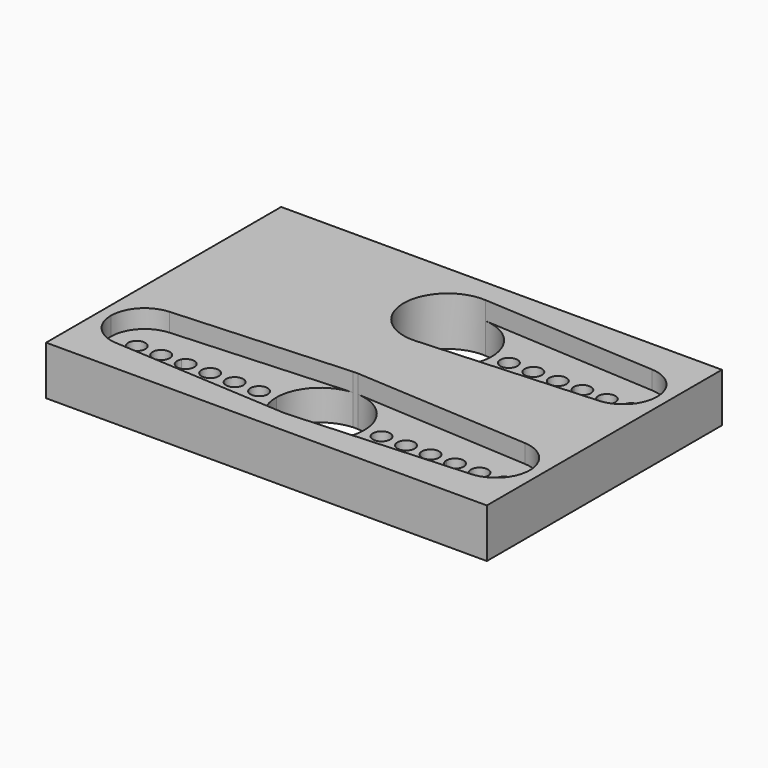
from build123d import *

# Parameters (mm, degrees)
F1_DEPTH = 4
F2_DEPTH = 1.5


with BuildPart() as f1:
    # F0 (on Top) → F1 (new body)
    with BuildSketch(Plane.XY):
        with BuildLine():
            Line((18, 12), (-18, 12))
            Line((-18, 12), (-18, -6.5))
            Line((-18, -6.5), (-17.1, -6.5))
            ThreePointArc((-17.1, -6.5), (-16.3513061937, -4.613926428), (-14.5128919861, -3.7548285662))
            Line((-14.5128919861, -3.7548285662), (-0.2132404181, -2.9063210321))
            ThreePointArc((-0.2132404181, -2.9063210321), (0, -2.9), (0.2132404181, -2.9063210321))
            Line((0.2132404181, -2.9063210321), (14.5128919861, -3.7548285662))
            ThreePointArc((14.5128919861, -3.7548285662), (16.3513061937, -4.613926428), (17.1, -6.5))
            Line((17.1, -6.5), (18, -6.5))
            Line((18, -6.5), (18, 6.5))
            Line((18, 6.5), (18, 12))
        make_face()
        with BuildLine():
            ThreePointArc((14.5128919861, 9.2451714338), (16.3513061937, 8.386073572), (17.1, 6.5))
            ThreePointArc((17.1, 6.5), (16.3513061937, 4.613926428), (14.5128919861, 3.7548285662))
            Line((14.5128919861, 3.7548285662), (0.2132404181, 2.9063210321))
            ThreePointArc((0.2132404181, 2.9063210321), (-3.6, 6.5), (0.2132404181, 10.0936789679))
            Line((0.2132404181, 10.0936789679), (14.5128919861, 9.2451714338))
        make_face(mode=Mode.SUBTRACT)
        with BuildLine():
            Line((-17.1, -6.5), (-18, -6.5))
            Line((-18, -6.5), (-18, -12))
            Line((-18, -12), (18, -12))
            Line((18, -12), (18, -6.5))
            Line((18, -6.5), (17.1, -6.5))
            ThreePointArc((17.1, -6.5), (16.3513061937, -8.386073572), (14.5128919861, -9.2451714338))
            Line((14.5128919861, -9.2451714338), (0.2132404181, -10.0936789679))
            ThreePointArc((0.2132404181, -10.0936789679), (0, -10.1), (-0.2132404181, -10.0936789679))
            Line((-0.2132404181, -10.0936789679), (-14.5128919861, -9.2451714338))
            ThreePointArc((-14.5128919861, -9.2451714338), (-16.3513061937, -8.386073572), (-17.1, -6.5))
        make_face()
        with BuildLine():
            ThreePointArc((-14.5128919861, -3.7548285662), (-16.3513061937, -4.613926428), (-17.1, -6.5))
            Line((-17.1, -6.5), (-15.7, -6.5))
            ThreePointArc((-15.7, -6.5), (-15, -5.8), (-14.3, -6.5))
            Line((-14.3, -6.5), (-13.7, -6.5))
            ThreePointArc((-13.7, -6.5), (-13, -5.8), (-12.3, -6.5))
            Line((-12.3, -6.5), (-11.7, -6.5))
            ThreePointArc((-11.7, -6.5), (-11.6795520913, -6.3320447821), (-11.6194029851, -6.1739019441))
            ThreePointArc((-11.6194029851, -6.1739019441), (-12.5861246414, -4.3902029199), (-14.5128919861, -3.7548285662))
        make_face()
        with BuildLine():
            Line((-15.7, -6.5), (-17.1, -6.5))
            ThreePointArc((-17.1, -6.5), (-16.3513061937, -8.386073572), (-14.5128919861, -9.2451714338))
            ThreePointArc((-14.5128919861, -9.2451714338), (-12.5861246414, -8.6097970801), (-11.6194029851, -6.8260980559))
            ThreePointArc((-11.6194029851, -6.8260980559), (-11.6795520913, -6.6679552179), (-11.7, -6.5))
            Line((-11.7, -6.5), (-12.3, -6.5))
            ThreePointArc((-12.3, -6.5), (-13, -7.2), (-13.7, -6.5))
            Line((-13.7, -6.5), (-14.3, -6.5))
            ThreePointArc((-14.3, -6.5), (-15, -7.2), (-15.7, -6.5))
        make_face()
        with BuildLine():
            Line((-0.2132404181, -2.9063210321), (-14.5128919861, -3.7548285662))
            ThreePointArc((-14.5128919861, -3.7548285662), (-12.5861246414, -4.3902029199), (-11.6194029851, -6.1739019441))
            ThreePointArc((-11.6194029851, -6.1739019441), (-10.8320447821, -5.8204479087), (-10.3, -6.5))
            Line((-10.3, -6.5), (-9.7, -6.5))
            ThreePointArc((-9.7, -6.5), (-9, -5.8), (-8.3, -6.5))
            Line((-8.3, -6.5), (-7.7, -6.5))
            ThreePointArc((-7.7, -6.5), (-7, -5.8), (-6.3, -6.5))
            Line((-6.3, -6.5), (-5.7, -6.5))
            ThreePointArc((-5.7, -6.5), (-5, -5.8), (-4.3, -6.5))
            Line((-4.3, -6.5), (-3.6, -6.5))
            ThreePointArc((-3.6, -6.5), (-2.6198917444, -4.030958233), (-0.2132404181, -2.9063210321))
        make_face()
        with BuildLine():
            ThreePointArc((-11.6194029851, -6.8260980559), (-12.5861246414, -8.6097970801), (-14.5128919861, -9.2451714338))
            Line((-14.5128919861, -9.2451714338), (-0.2132404181, -10.0936789679))
            ThreePointArc((-0.2132404181, -10.0936789679), (-2.6198917444, -8.969041767), (-3.6, -6.5))
            Line((-3.6, -6.5), (-4.3, -6.5))
            ThreePointArc((-4.3, -6.5), (-5, -7.2), (-5.7, -6.5))
            Line((-5.7, -6.5), (-6.3, -6.5))
            ThreePointArc((-6.3, -6.5), (-7, -7.2), (-7.7, -6.5))
            Line((-7.7, -6.5), (-8.3, -6.5))
            ThreePointArc((-8.3, -6.5), (-9, -7.2), (-9.7, -6.5))
            Line((-9.7, -6.5), (-10.3, -6.5))
            ThreePointArc((-10.3, -6.5), (-10.8320447821, -7.1795520913), (-11.6194029851, -6.8260980559))
        make_face()
        with BuildLine():
            Line((0.2132404181, -10.0936789679), (14.5128919861, -9.2451714338))
            ThreePointArc((14.5128919861, -9.2451714338), (12.5861246414, -8.6097970801), (11.6194029851, -6.8260980559))
            ThreePointArc((11.6194029851, -6.8260980559), (10.8320447821, -7.1795520913), (10.3, -6.5))
            Line((10.3, -6.5), (9.7, -6.5))
            ThreePointArc((9.7, -6.5), (9, -7.2), (8.3, -6.5))
            Line((8.3, -6.5), (7.7, -6.5))
            ThreePointArc((7.7, -6.5), (7, -7.2), (6.3, -6.5))
            Line((6.3, -6.5), (5.7, -6.5))
            ThreePointArc((5.7, -6.5), (5, -7.2), (4.3, -6.5))
            Line((4.3, -6.5), (3.6, -6.5))
            ThreePointArc((3.6, -6.5), (2.6198917444, -8.969041767), (0.2132404181, -10.0936789679))
        make_face()
        with BuildLine():
            ThreePointArc((11.6194029851, -6.1739019441), (12.5861246414, -4.3902029199), (14.5128919861, -3.7548285662))
            Line((14.5128919861, -3.7548285662), (0.2132404181, -2.9063210321))
            ThreePointArc((0.2132404181, -2.9063210321), (2.6198917444, -4.030958233), (3.6, -6.5))
            Line((3.6, -6.5), (4.3, -6.5))
            ThreePointArc((4.3, -6.5), (5, -5.8), (5.7, -6.5))
            Line((5.7, -6.5), (6.3, -6.5))
            ThreePointArc((6.3, -6.5), (7, -5.8), (7.7, -6.5))
            Line((7.7, -6.5), (8.3, -6.5))
            ThreePointArc((8.3, -6.5), (9, -5.8), (9.7, -6.5))
            Line((9.7, -6.5), (10.3, -6.5))
            ThreePointArc((10.3, -6.5), (10.8320447821, -5.8204479087), (11.6194029851, -6.1739019441))
        make_face()
        with BuildLine():
            Line((0.2132404181, 2.9063210321), (14.5128919861, 3.7548285662))
            ThreePointArc((14.5128919861, 3.7548285662), (12.5861246414, 4.3902029199), (11.6194029851, 6.1739019441))
            ThreePointArc((11.6194029851, 6.1739019441), (10.8320447821, 5.8204479087), (10.3, 6.5))
            Line((10.3, 6.5), (9.7, 6.5))
            ThreePointArc((9.7, 6.5), (9, 5.8), (8.3, 6.5))
            Line((8.3, 6.5), (7.7, 6.5))
            ThreePointArc((7.7, 6.5), (7, 5.8), (6.3, 6.5))
            Line((6.3, 6.5), (5.7, 6.5))
            ThreePointArc((5.7, 6.5), (5, 5.8), (4.3, 6.5))
            Line((4.3, 6.5), (3.6, 6.5))
            ThreePointArc((3.6, 6.5), (2.6198917444, 4.030958233), (0.2132404181, 2.9063210321))
        make_face()
        with BuildLine():
            ThreePointArc((11.6194029851, 6.8260980559), (12.5861246414, 8.6097970801), (14.5128919861, 9.2451714338))
            Line((14.5128919861, 9.2451714338), (0.2132404181, 10.0936789679))
            ThreePointArc((0.2132404181, 10.0936789679), (2.6198917444, 8.969041767), (3.6, 6.5))
            Line((3.6, 6.5), (4.3, 6.5))
            ThreePointArc((4.3, 6.5), (5, 7.2), (5.7, 6.5))
            Line((5.7, 6.5), (6.3, 6.5))
            ThreePointArc((6.3, 6.5), (7, 7.2), (7.7, 6.5))
            Line((7.7, 6.5), (8.3, 6.5))
            ThreePointArc((8.3, 6.5), (9, 7.2), (9.7, 6.5))
            Line((9.7, 6.5), (10.3, 6.5))
            ThreePointArc((10.3, 6.5), (10.8320447821, 7.1795520913), (11.6194029851, 6.8260980559))
        make_face()
        with BuildLine():
            ThreePointArc((14.5128919861, 3.7548285662), (16.3513061937, 4.613926428), (17.1, 6.5))
            Line((17.1, 6.5), (15.7, 6.5))
            ThreePointArc((15.7, 6.5), (15, 5.8), (14.3, 6.5))
            Line((14.3, 6.5), (13.7, 6.5))
            ThreePointArc((13.7, 6.5), (13, 5.8), (12.3, 6.5))
            Line((12.3, 6.5), (11.7, 6.5))
            ThreePointArc((11.7, 6.5), (11.6795520913, 6.3320447821), (11.6194029851, 6.1739019441))
            ThreePointArc((11.6194029851, 6.1739019441), (12.5861246414, 4.3902029199), (14.5128919861, 3.7548285662))
        make_face()
        with BuildLine():
            Line((15.7, 6.5), (17.1, 6.5))
            ThreePointArc((17.1, 6.5), (16.3513061937, 8.386073572), (14.5128919861, 9.2451714338))
            ThreePointArc((14.5128919861, 9.2451714338), (12.5861246414, 8.6097970801), (11.6194029851, 6.8260980559))
            ThreePointArc((11.6194029851, 6.8260980559), (11.6795520913, 6.6679552179), (11.7, 6.5))
            Line((11.7, 6.5), (12.3, 6.5))
            ThreePointArc((12.3, 6.5), (13, 7.2), (13.7, 6.5))
            Line((13.7, 6.5), (14.3, 6.5))
            ThreePointArc((14.3, 6.5), (15, 7.2), (15.7, 6.5))
        make_face()
        with BuildLine():
            Line((15.7, -6.5), (17.1, -6.5))
            ThreePointArc((17.1, -6.5), (16.3513061937, -4.613926428), (14.5128919861, -3.7548285662))
            ThreePointArc((14.5128919861, -3.7548285662), (12.5861246414, -4.3902029199), (11.6194029851, -6.1739019441))
            ThreePointArc((11.6194029851, -6.1739019441), (11.6795520913, -6.3320447821), (11.7, -6.5))
            Line((11.7, -6.5), (12.3, -6.5))
            ThreePointArc((12.3, -6.5), (13, -5.8), (13.7, -6.5))
            Line((13.7, -6.5), (14.3, -6.5))
            ThreePointArc((14.3, -6.5), (15, -5.8), (15.7, -6.5))
        make_face()
        with BuildLine():
            ThreePointArc((14.5128919861, -9.2451714338), (16.3513061937, -8.386073572), (17.1, -6.5))
            Line((17.1, -6.5), (15.7, -6.5))
            ThreePointArc((15.7, -6.5), (15, -7.2), (14.3, -6.5))
            Line((14.3, -6.5), (13.7, -6.5))
            ThreePointArc((13.7, -6.5), (13, -7.2), (12.3, -6.5))
            Line((12.3, -6.5), (11.7, -6.5))
            ThreePointArc((11.7, -6.5), (11.6795520913, -6.6679552179), (11.6194029851, -6.8260980559))
            ThreePointArc((11.6194029851, -6.8260980559), (12.5861246414, -8.6097970801), (14.5128919861, -9.2451714338))
        make_face()
    extrude(amount=-F1_DEPTH)

    # F0 (on Top) → F2 (cut)
    with BuildSketch(Plane.XY):
        with BuildLine():
            ThreePointArc((14.5128919861, 3.7548285662), (16.3513061937, 4.613926428), (17.1, 6.5))
            Line((17.1, 6.5), (15.7, 6.5))
            ThreePointArc((15.7, 6.5), (15, 5.8), (14.3, 6.5))
            Line((14.3, 6.5), (13.7, 6.5))
            ThreePointArc((13.7, 6.5), (13, 5.8), (12.3, 6.5))
            Line((12.3, 6.5), (11.7, 6.5))
            ThreePointArc((11.7, 6.5), (11.6795520913, 6.3320447821), (11.6194029851, 6.1739019441))
            ThreePointArc((11.6194029851, 6.1739019441), (12.5861246414, 4.3902029199), (14.5128919861, 3.7548285662))
        make_face()
        with BuildLine():
            Line((15.7, 6.5), (17.1, 6.5))
            ThreePointArc((17.1, 6.5), (16.3513061937, 8.386073572), (14.5128919861, 9.2451714338))
            ThreePointArc((14.5128919861, 9.2451714338), (12.5861246414, 8.6097970801), (11.6194029851, 6.8260980559))
            ThreePointArc((11.6194029851, 6.8260980559), (11.6795520913, 6.6679552179), (11.7, 6.5))
            Line((11.7, 6.5), (12.3, 6.5))
            ThreePointArc((12.3, 6.5), (13, 7.2), (13.7, 6.5))
            Line((13.7, 6.5), (14.3, 6.5))
            ThreePointArc((14.3, 6.5), (15, 7.2), (15.7, 6.5))
        make_face()
        with BuildLine():
            ThreePointArc((-14.5128919861, -3.7548285662), (-16.3513061937, -4.613926428), (-17.1, -6.5))
            Line((-17.1, -6.5), (-15.7, -6.5))
            ThreePointArc((-15.7, -6.5), (-15, -5.8), (-14.3, -6.5))
            Line((-14.3, -6.5), (-13.7, -6.5))
            ThreePointArc((-13.7, -6.5), (-13, -5.8), (-12.3, -6.5))
            Line((-12.3, -6.5), (-11.7, -6.5))
            ThreePointArc((-11.7, -6.5), (-11.6795520913, -6.3320447821), (-11.6194029851, -6.1739019441))
            ThreePointArc((-11.6194029851, -6.1739019441), (-12.5861246414, -4.3902029199), (-14.5128919861, -3.7548285662))
        make_face()
        with BuildLine():
            Line((-15.7, -6.5), (-17.1, -6.5))
            ThreePointArc((-17.1, -6.5), (-16.3513061937, -8.386073572), (-14.5128919861, -9.2451714338))
            ThreePointArc((-14.5128919861, -9.2451714338), (-12.5861246414, -8.6097970801), (-11.6194029851, -6.8260980559))
            ThreePointArc((-11.6194029851, -6.8260980559), (-11.6795520913, -6.6679552179), (-11.7, -6.5))
            Line((-11.7, -6.5), (-12.3, -6.5))
            ThreePointArc((-12.3, -6.5), (-13, -7.2), (-13.7, -6.5))
            Line((-13.7, -6.5), (-14.3, -6.5))
            ThreePointArc((-14.3, -6.5), (-15, -7.2), (-15.7, -6.5))
        make_face()
        with BuildLine():
            Line((-0.2132404181, -2.9063210321), (-14.5128919861, -3.7548285662))
            ThreePointArc((-14.5128919861, -3.7548285662), (-12.5861246414, -4.3902029199), (-11.6194029851, -6.1739019441))
            ThreePointArc((-11.6194029851, -6.1739019441), (-10.8320447821, -5.8204479087), (-10.3, -6.5))
            Line((-10.3, -6.5), (-9.7, -6.5))
            ThreePointArc((-9.7, -6.5), (-9, -5.8), (-8.3, -6.5))
            Line((-8.3, -6.5), (-7.7, -6.5))
            ThreePointArc((-7.7, -6.5), (-7, -5.8), (-6.3, -6.5))
            Line((-6.3, -6.5), (-5.7, -6.5))
            ThreePointArc((-5.7, -6.5), (-5, -5.8), (-4.3, -6.5))
            Line((-4.3, -6.5), (-3.6, -6.5))
            ThreePointArc((-3.6, -6.5), (-2.6198917444, -4.030958233), (-0.2132404181, -2.9063210321))
        make_face()
        with BuildLine():
            ThreePointArc((-11.6194029851, -6.8260980559), (-12.5861246414, -8.6097970801), (-14.5128919861, -9.2451714338))
            Line((-14.5128919861, -9.2451714338), (-0.2132404181, -10.0936789679))
            ThreePointArc((-0.2132404181, -10.0936789679), (-2.6198917444, -8.969041767), (-3.6, -6.5))
            Line((-3.6, -6.5), (-4.3, -6.5))
            ThreePointArc((-4.3, -6.5), (-5, -7.2), (-5.7, -6.5))
            Line((-5.7, -6.5), (-6.3, -6.5))
            ThreePointArc((-6.3, -6.5), (-7, -7.2), (-7.7, -6.5))
            Line((-7.7, -6.5), (-8.3, -6.5))
            ThreePointArc((-8.3, -6.5), (-9, -7.2), (-9.7, -6.5))
            Line((-9.7, -6.5), (-10.3, -6.5))
            ThreePointArc((-10.3, -6.5), (-10.8320447821, -7.1795520913), (-11.6194029851, -6.8260980559))
        make_face()
        with BuildLine():
            ThreePointArc((14.5128919861, -9.2451714338), (16.3513061937, -8.386073572), (17.1, -6.5))
            Line((17.1, -6.5), (15.7, -6.5))
            ThreePointArc((15.7, -6.5), (15, -7.2), (14.3, -6.5))
            Line((14.3, -6.5), (13.7, -6.5))
            ThreePointArc((13.7, -6.5), (13, -7.2), (12.3, -6.5))
            Line((12.3, -6.5), (11.7, -6.5))
            ThreePointArc((11.7, -6.5), (11.6795520913, -6.6679552179), (11.6194029851, -6.8260980559))
            ThreePointArc((11.6194029851, -6.8260980559), (12.5861246414, -8.6097970801), (14.5128919861, -9.2451714338))
        make_face()
        with BuildLine():
            Line((15.7, -6.5), (17.1, -6.5))
            ThreePointArc((17.1, -6.5), (16.3513061937, -4.613926428), (14.5128919861, -3.7548285662))
            ThreePointArc((14.5128919861, -3.7548285662), (12.5861246414, -4.3902029199), (11.6194029851, -6.1739019441))
            ThreePointArc((11.6194029851, -6.1739019441), (11.6795520913, -6.3320447821), (11.7, -6.5))
            Line((11.7, -6.5), (12.3, -6.5))
            ThreePointArc((12.3, -6.5), (13, -5.8), (13.7, -6.5))
            Line((13.7, -6.5), (14.3, -6.5))
            ThreePointArc((14.3, -6.5), (15, -5.8), (15.7, -6.5))
        make_face()
        with BuildLine():
            ThreePointArc((11.6194029851, 6.8260980559), (12.5861246414, 8.6097970801), (14.5128919861, 9.2451714338))
            Line((14.5128919861, 9.2451714338), (0.2132404181, 10.0936789679))
            ThreePointArc((0.2132404181, 10.0936789679), (2.6198917444, 8.969041767), (3.6, 6.5))
            Line((3.6, 6.5), (4.3, 6.5))
            ThreePointArc((4.3, 6.5), (5, 7.2), (5.7, 6.5))
            Line((5.7, 6.5), (6.3, 6.5))
            ThreePointArc((6.3, 6.5), (7, 7.2), (7.7, 6.5))
            Line((7.7, 6.5), (8.3, 6.5))
            ThreePointArc((8.3, 6.5), (9, 7.2), (9.7, 6.5))
            Line((9.7, 6.5), (10.3, 6.5))
            ThreePointArc((10.3, 6.5), (10.8320447821, 7.1795520913), (11.6194029851, 6.8260980559))
        make_face()
        with BuildLine():
            Line((0.2132404181, 2.9063210321), (14.5128919861, 3.7548285662))
            ThreePointArc((14.5128919861, 3.7548285662), (12.5861246414, 4.3902029199), (11.6194029851, 6.1739019441))
            ThreePointArc((11.6194029851, 6.1739019441), (10.8320447821, 5.8204479087), (10.3, 6.5))
            Line((10.3, 6.5), (9.7, 6.5))
            ThreePointArc((9.7, 6.5), (9, 5.8), (8.3, 6.5))
            Line((8.3, 6.5), (7.7, 6.5))
            ThreePointArc((7.7, 6.5), (7, 5.8), (6.3, 6.5))
            Line((6.3, 6.5), (5.7, 6.5))
            ThreePointArc((5.7, 6.5), (5, 5.8), (4.3, 6.5))
            Line((4.3, 6.5), (3.6, 6.5))
            ThreePointArc((3.6, 6.5), (2.6198917444, 4.030958233), (0.2132404181, 2.9063210321))
        make_face()
        with BuildLine():
            ThreePointArc((11.6194029851, -6.1739019441), (12.5861246414, -4.3902029199), (14.5128919861, -3.7548285662))
            Line((14.5128919861, -3.7548285662), (0.2132404181, -2.9063210321))
            ThreePointArc((0.2132404181, -2.9063210321), (2.6198917444, -4.030958233), (3.6, -6.5))
            Line((3.6, -6.5), (4.3, -6.5))
            ThreePointArc((4.3, -6.5), (5, -5.8), (5.7, -6.5))
            Line((5.7, -6.5), (6.3, -6.5))
            ThreePointArc((6.3, -6.5), (7, -5.8), (7.7, -6.5))
            Line((7.7, -6.5), (8.3, -6.5))
            ThreePointArc((8.3, -6.5), (9, -5.8), (9.7, -6.5))
            Line((9.7, -6.5), (10.3, -6.5))
            ThreePointArc((10.3, -6.5), (10.8320447821, -5.8204479087), (11.6194029851, -6.1739019441))
        make_face()
        with BuildLine():
            Line((0.2132404181, -10.0936789679), (14.5128919861, -9.2451714338))
            ThreePointArc((14.5128919861, -9.2451714338), (12.5861246414, -8.6097970801), (11.6194029851, -6.8260980559))
            ThreePointArc((11.6194029851, -6.8260980559), (10.8320447821, -7.1795520913), (10.3, -6.5))
            Line((10.3, -6.5), (9.7, -6.5))
            ThreePointArc((9.7, -6.5), (9, -7.2), (8.3, -6.5))
            Line((8.3, -6.5), (7.7, -6.5))
            ThreePointArc((7.7, -6.5), (7, -7.2), (6.3, -6.5))
            Line((6.3, -6.5), (5.7, -6.5))
            ThreePointArc((5.7, -6.5), (5, -7.2), (4.3, -6.5))
            Line((4.3, -6.5), (3.6, -6.5))
            ThreePointArc((3.6, -6.5), (2.6198917444, -8.969041767), (0.2132404181, -10.0936789679))
        make_face()
        with BuildLine():
            ThreePointArc((11.7, 6.5), (11.6795520913, 6.6679552179), (11.6194029851, 6.8260980559))
            ThreePointArc((11.6194029851, 6.8260980559), (11.604855032, 6.6633373946), (11.6, 6.5))
            Line((11.6, 6.5), (11.7, 6.5))
        make_face()
        with BuildLine():
            ThreePointArc((11.6, 6.5), (11.604855032, 6.3366626054), (11.6194029851, 6.1739019441))
            ThreePointArc((11.6194029851, 6.1739019441), (11.6795520913, 6.3320447821), (11.7, 6.5))
            Line((11.7, 6.5), (11.6, 6.5))
        make_face()
    extrude(amount=-F2_DEPTH, mode=Mode.SUBTRACT)


solid = f1.part
